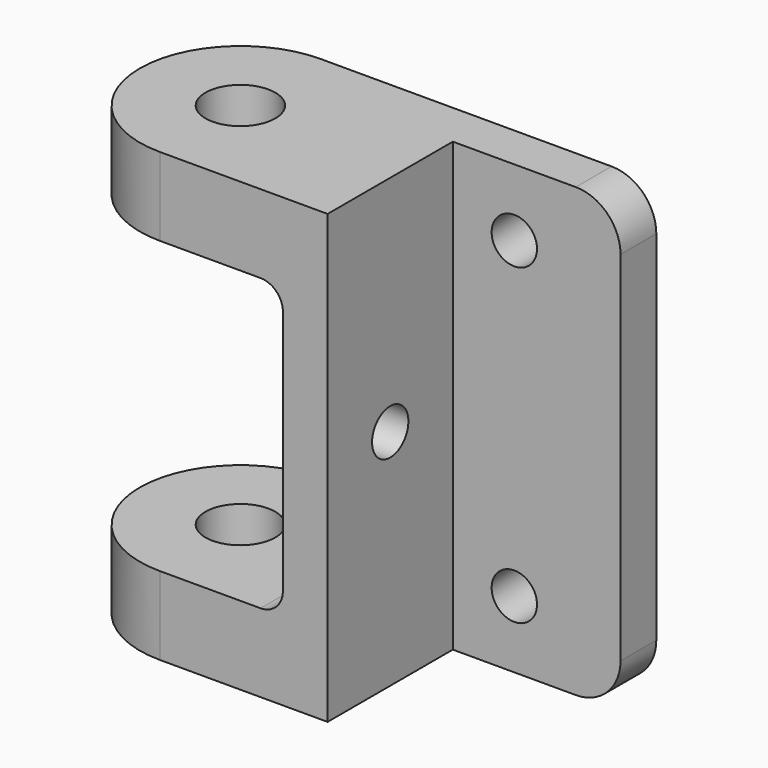
from build123d import *

# Parameters (mm, degrees)
F0_W      = 99.06
F0_H      = 101.6
F1_DEPTH  = 45.72
F2_W      = 45.8418870593
F2_H      = 107.1278404426
F3_DEPTH  = 35.56
F4_W      = 96.4650140689
F4_H      = 66.04
F5_DEPTH  = 45.721
F6_R      = 22.85999
F7_R      = 7.9375
F8_DEPTH  = 101.601
F9_R      = 5.08
F10_R     = 10.16
F11_R     = 5.1562
F12_DEPTH = 60.961
F13_R     = 5.1562
F14_DEPTH = 10.161


# Not quite as in the source:
# - a fillet or chamfer is up to 0.001 mm smaller than in the source, because OpenCascade refuses the exact size


with BuildPart() as f1:
    # F0 (on Front) → F1 (new body)
    with BuildSketch(Plane.XZ):
        with Locations((5.5195279419, -10.1849297343)):
            Rectangle(F0_W, F0_H)
    extrude(amount=F1_DEPTH)

    # F2 (on face) → F3 (cut)
    with BuildSketch(Plane.XZ.offset(45.72)):
        with Locations((39.8704714716, -9.8085980862)):
            Rectangle(F2_W, F2_H)
    extrude(amount=-F3_DEPTH, mode=Mode.SUBTRACT)

    # F4 (on face) → F5 (cut, through all)
    with BuildSketch(Plane.XZ.offset(45.72)):
        with Locations((-41.4429790925, -10.1849297343)):
            Rectangle(F4_W, F4_H)
    extrude(amount=-F5_DEPTH, mode=Mode.SUBTRACT)

    # F6 (radius 22.86 in the source; OpenCascade refuses exactly that, so slightly less here)
    f6_edges = [f1.edges().sort_by_distance(p)[0] for p in [
        (-44.010472, 0, 31.72507),
        (-44.010472, -45.72, 31.72507),
        (-44.010472, 0, -52.09493),
        (-44.010472, -45.72, -52.09493),
    ]]
    fillet(f6_edges, radius=F6_R)

    # F7 (on face) → F8 (cut, through all)
    with BuildSketch(Plane.XY.offset(40.6150702657)):
        with Locations((-21.1504720581, -22.86)):
            Circle(F7_R)
    extrude(amount=-F8_DEPTH, mode=Mode.SUBTRACT)

    # F9
    f9_edges = [f1.edges().sort_by_distance(p)[0] for p in [
        (6.789528, -22.86, 22.83507),
        (6.789528, -22.86, -43.20493),
    ]]
    fillet(f9_edges, radius=F9_R)

    # F10
    f10_edges = [f1.edges().sort_by_distance(p)[0] for p in [
        (55.049528, -5.08, 40.61507),
        (55.049528, -5.08, -60.98493),
    ]]
    fillet(f10_edges, radius=F10_R)

    # F11 (on face) → F12 (cut, through all)
    with BuildSketch(Plane.YZ.offset(16.9495279419)):
        with Locations((-27.94, -10.1849297343)):
            Circle(F11_R)
    extrude(amount=-F12_DEPTH, mode=Mode.SUBTRACT)

    # F13 (on face) → F14 (cut, through all)
    with BuildSketch(Plane.XZ.offset(10.16)):
        with Locations((30.9195279419, 25.3750702657)):
            Circle(F13_R)
        with Locations((30.9195279419, -45.7449297343)):
            Circle(F13_R)
    extrude(amount=-F14_DEPTH, mode=Mode.SUBTRACT)


solid = f1.part
